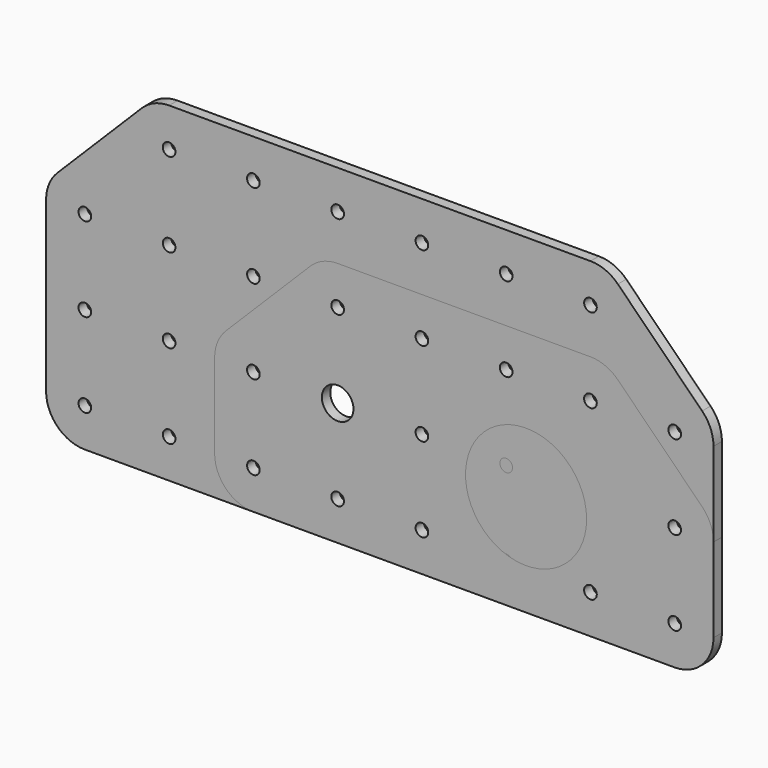
from build123d import *

# Parameters (mm, degrees)
F0_R     = 1.905
F0_R_2   = 4.7625
F0_R_3   = 6.604
F1_DEPTH = 3.175
F2_R     = 1.905
F2_R_2   = 4.7625
F3_DEPTH = 3.175
F4_R     = 1.905
F4_R_2   = 18.2499
F4_R_3   = 4.7625
F5_DEPTH = 3.175
F6_R     = 11.684
F6_2_R   = 11.684
F6_3_R   = 11.684


# Not quite as in the source:
# - a feature names something its author has since deleted; it is built from what else it names


with BuildPart() as f1:
    # F0 (on Front) → F1 (new body)
    with BuildSketch(Plane.XZ):
        Polygon((-87.884, 30.2396712628), (-87.884, -37.084), (113.284, -37.084), (113.284, 30.2396712628), (81.0396712628, 62.484), (-55.6396712628, 62.484), align=None)
        with Locations((-76.2, -25.4)):
            Circle(F0_R, mode=Mode.SUBTRACT)
        with Locations((-50.8, -25.4)):
            Circle(F0_R, mode=Mode.SUBTRACT)
        with Locations((-25.4, -25.4)):
            Circle(F0_R, mode=Mode.SUBTRACT)
        with Locations((0, -25.4)):
            Circle(F0_R, mode=Mode.SUBTRACT)
        with Locations((-76.2, 0)):
            Circle(F0_R, mode=Mode.SUBTRACT)
        with Locations((-50.8, 0)):
            Circle(F0_R, mode=Mode.SUBTRACT)
        with Locations((-25.4, 0)):
            Circle(F0_R, mode=Mode.SUBTRACT)
        Circle(F0_R_2, mode=Mode.SUBTRACT)
        with Locations((25.4, -25.4)):
            Circle(F0_R, mode=Mode.SUBTRACT)
        with Locations((56.7918539792, -18.8849)):
            Circle(F0_R, mode=Mode.SUBTRACT)
        with Locations((76.2, -25.4)):
            Circle(F0_R, mode=Mode.SUBTRACT)
        with Locations((101.6, -25.4)):
            Circle(F0_R, mode=Mode.SUBTRACT)
        with Locations((25.4, 0)):
            Circle(F0_R, mode=Mode.SUBTRACT)
        with Locations((56.7918539792, -6.3881)):
            Circle(F0_R_3, mode=Mode.SUBTRACT)
        with Locations((56.7918539792, 6.1087)):
            Circle(F0_R, mode=Mode.SUBTRACT)
        with Locations((76.2, 0)):
            Circle(F0_R, mode=Mode.SUBTRACT)
        with Locations((101.6, 0)):
            Circle(F0_R, mode=Mode.SUBTRACT)
        with Locations((-76.2, 25.4)):
            Circle(F0_R, mode=Mode.SUBTRACT)
        with Locations((-50.8, 25.4)):
            Circle(F0_R, mode=Mode.SUBTRACT)
        with Locations((-25.4, 25.4)):
            Circle(F0_R, mode=Mode.SUBTRACT)
        with Locations((0, 25.4)):
            Circle(F0_R, mode=Mode.SUBTRACT)
        with Locations((-50.8, 50.8)):
            Circle(F0_R, mode=Mode.SUBTRACT)
        with Locations((-25.4, 50.8)):
            Circle(F0_R, mode=Mode.SUBTRACT)
        with Locations((0, 50.8)):
            Circle(F0_R, mode=Mode.SUBTRACT)
        with Locations((25.4, 25.4)):
            Circle(F0_R, mode=Mode.SUBTRACT)
        with Locations((50.8, 25.4)):
            Circle(F0_R, mode=Mode.SUBTRACT)
        with Locations((76.2, 25.4)):
            Circle(F0_R, mode=Mode.SUBTRACT)
        with Locations((101.6, 25.4)):
            Circle(F0_R, mode=Mode.SUBTRACT)
        with Locations((25.4, 50.8)):
            Circle(F0_R, mode=Mode.SUBTRACT)
        with Locations((50.8, 50.8)):
            Circle(F0_R, mode=Mode.SUBTRACT)
        with Locations((76.2, 50.8)):
            Circle(F0_R, mode=Mode.SUBTRACT)
    extrude(amount=F1_DEPTH)

    # F6#2
    f6_2_edges = [f1.edges().sort_by_distance(p)[0] for p in [
        (-87.884, -1.5875, 30.239671),
        (-55.639671, -1.5875, 62.484),
        (81.039671, -1.5875, 62.484),
        (113.284, -1.5875, 30.239671),
        (113.284, -1.5875, -37.084),
        (-87.884, -1.5875, -37.084),
    ]]
    fillet(f6_2_edges, radius=F6_2_R)


with BuildPart() as f3:
    # F2 (on Front) → F3 (new body)
    with BuildSketch(Plane.XZ):
        Polygon((-87.884, 30.2396712628), (-87.884, -37.084), (113.284, -37.084), (113.284, 30.2396712628), (81.0396712628, 62.484), (-55.6396712628, 62.484), align=None)
        with Locations((-76.2, -25.4)):
            Circle(F2_R, mode=Mode.SUBTRACT)
        with Locations((-50.8, -25.4)):
            Circle(F2_R, mode=Mode.SUBTRACT)
        with Locations((-25.4, -25.4)):
            Circle(F2_R, mode=Mode.SUBTRACT)
        with Locations((0, -25.4)):
            Circle(F2_R, mode=Mode.SUBTRACT)
        with Locations((-76.2, 0)):
            Circle(F2_R, mode=Mode.SUBTRACT)
        with Locations((-50.8, 0)):
            Circle(F2_R, mode=Mode.SUBTRACT)
        with Locations((-25.4, 0)):
            Circle(F2_R, mode=Mode.SUBTRACT)
        Circle(F2_R_2, mode=Mode.SUBTRACT)
        with Locations((25.4, -25.4)):
            Circle(F2_R, mode=Mode.SUBTRACT)
        with Locations((50.8, -25.4)):
            Circle(F2_R, mode=Mode.SUBTRACT)
        with Locations((76.2, -25.4)):
            Circle(F2_R, mode=Mode.SUBTRACT)
        with Locations((101.6, -25.4)):
            Circle(F2_R, mode=Mode.SUBTRACT)
        with Locations((25.4, 0)):
            Circle(F2_R, mode=Mode.SUBTRACT)
        with Locations((50.8, 0)):
            Circle(F2_R, mode=Mode.SUBTRACT)
        with Locations((76.2, 0)):
            Circle(F2_R, mode=Mode.SUBTRACT)
        with Locations((101.6, 0)):
            Circle(F2_R, mode=Mode.SUBTRACT)
        with Locations((-76.2, 25.4)):
            Circle(F2_R, mode=Mode.SUBTRACT)
        with Locations((-50.8, 25.4)):
            Circle(F2_R, mode=Mode.SUBTRACT)
        with Locations((-25.4, 25.4)):
            Circle(F2_R, mode=Mode.SUBTRACT)
        with Locations((0, 25.4)):
            Circle(F2_R, mode=Mode.SUBTRACT)
        with Locations((-50.8, 50.8)):
            Circle(F2_R, mode=Mode.SUBTRACT)
        with Locations((-25.4, 50.8)):
            Circle(F2_R, mode=Mode.SUBTRACT)
        with Locations((0, 50.8)):
            Circle(F2_R, mode=Mode.SUBTRACT)
        with Locations((25.4, 25.4)):
            Circle(F2_R, mode=Mode.SUBTRACT)
        with Locations((50.8, 25.4)):
            Circle(F2_R, mode=Mode.SUBTRACT)
        with Locations((76.2, 25.4)):
            Circle(F2_R, mode=Mode.SUBTRACT)
        with Locations((101.6, 25.4)):
            Circle(F2_R, mode=Mode.SUBTRACT)
        with Locations((25.4, 50.8)):
            Circle(F2_R, mode=Mode.SUBTRACT)
        with Locations((50.8, 50.8)):
            Circle(F2_R, mode=Mode.SUBTRACT)
        with Locations((76.2, 50.8)):
            Circle(F2_R, mode=Mode.SUBTRACT)
    extrude(amount=F3_DEPTH)

    # F6
    f6_edges = [f3.edges().sort_by_distance(p)[0] for p in [
        (-87.884, -1.5875, 30.239671),
        (-55.639671, -1.5875, 62.484),
        (81.039671, -1.5875, 62.484),
        (113.284, -1.5875, 30.239671),
        (113.284, -1.5875, -37.084),
        (-87.884, -1.5875, -37.084),
    ]]
    fillet(f6_edges, radius=F6_R)


with BuildPart() as f5:
    # F4 (on Front) → F5 (new body)
    with BuildSketch(Plane.XZ):
        Polygon((-37.084, 4.8396712628), (-37.084, -37.084), (113.284, -37.084), (113.284, 4.8396712628), (81.0396712628, 37.084), (-4.8396712628, 37.084), align=None)
        with Locations((-25.4, -25.4)):
            Circle(F4_R, mode=Mode.SUBTRACT)
        with Locations((0, -25.4)):
            Circle(F4_R, mode=Mode.SUBTRACT)
        with Locations((25.4, -25.4)):
            Circle(F4_R, mode=Mode.SUBTRACT)
        with Locations((76.2, -25.4)):
            Circle(F4_R, mode=Mode.SUBTRACT)
        with Locations((101.6, -25.4)):
            Circle(F4_R, mode=Mode.SUBTRACT)
        with Locations((56.7918539792, -6.3881)):
            Circle(F4_R_2, mode=Mode.SUBTRACT)
        with Locations((-25.4, 0)):
            Circle(F4_R, mode=Mode.SUBTRACT)
        Circle(F4_R_3, mode=Mode.SUBTRACT)
        with Locations((25.4, 0)):
            Circle(F4_R, mode=Mode.SUBTRACT)
        with Locations((0, 25.4)):
            Circle(F4_R, mode=Mode.SUBTRACT)
        with Locations((25.4, 25.4)):
            Circle(F4_R, mode=Mode.SUBTRACT)
        with Locations((101.6, 0)):
            Circle(F4_R, mode=Mode.SUBTRACT)
        with Locations((50.8, 25.4)):
            Circle(F4_R, mode=Mode.SUBTRACT)
        with Locations((76.2, 25.4)):
            Circle(F4_R, mode=Mode.SUBTRACT)
    extrude(amount=F5_DEPTH)

    # F6#3
    f6_3_edges = [f5.edges().sort_by_distance(p)[0] for p in [
        (113.284, -1.5875, -37.084),
        (-37.084, -1.5875, -37.084),
        (-37.084, -1.5875, 4.839671),
        (-4.839671, -1.5875, 37.084),
        (81.039671, -1.5875, 37.084),
        (113.284, -1.5875, 4.839671),
    ]]
    fillet(f6_3_edges, radius=F6_3_R)


solid = Compound([f1.part, f3.part, f5.part])
